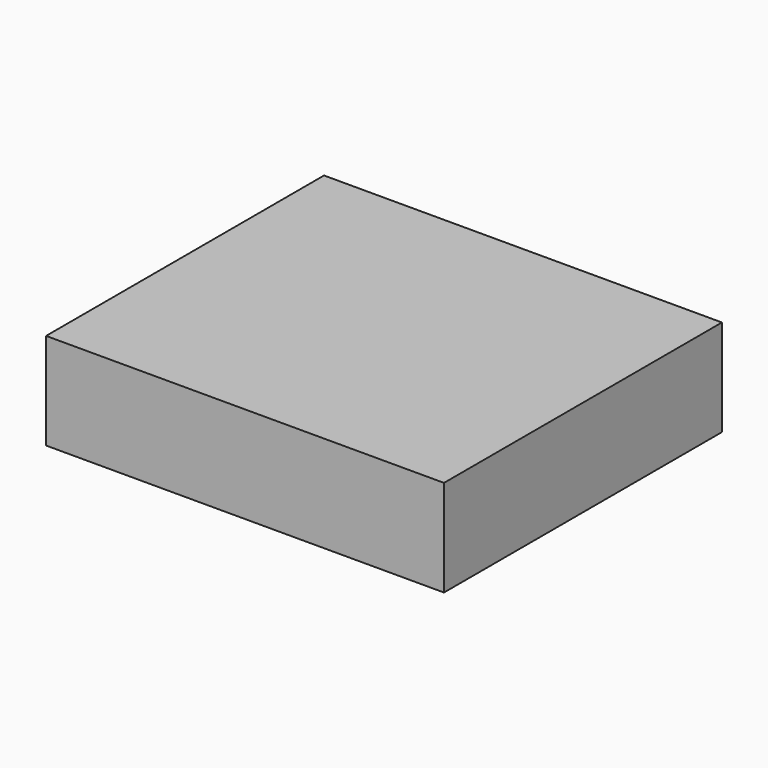
from build123d import *

# Parameters (mm, degrees)
F0_W     = 104.6971082687
F0_H     = 91.4116799831
F1_DEPTH = 25.4
F2_R     = 13.9798857956
F3_DEPTH = 25.4
F7_DEPTH = 127


# Not quite as in the source:
# - a feature of the source that left no trace in its solid (it failed there, or was rolled back) is left out


with BuildPart() as f1:
    # F0 (on Top) → F1 (new body)
    with BuildSketch(Plane.XY):
        Rectangle(F0_W, F0_H)
    extrude(amount=F1_DEPTH)

    # F2 (on face) → F3 (join)
    with BuildSketch(Plane(origin=(0, 0, 0), x_dir=(1, 0, 0), z_dir=(0, 0, -1))):
        Circle(F2_R)
    extrude(amount=F3_DEPTH)

    # F6 (on face) → F7 (cut)
    with BuildSketch(Plane(origin=(0, 45.7058399916, 0), x_dir=(-1, 0, 0), z_dir=(0, 1, 0))):
        Polygon((-14.2768789083, -25.4802610725), (13.8802975416, -25.4802610725), (-14.2768789083, -6.6427136771), align=None)
    extrude(amount=-F7_DEPTH, mode=Mode.SUBTRACT)


solid = f1.part
